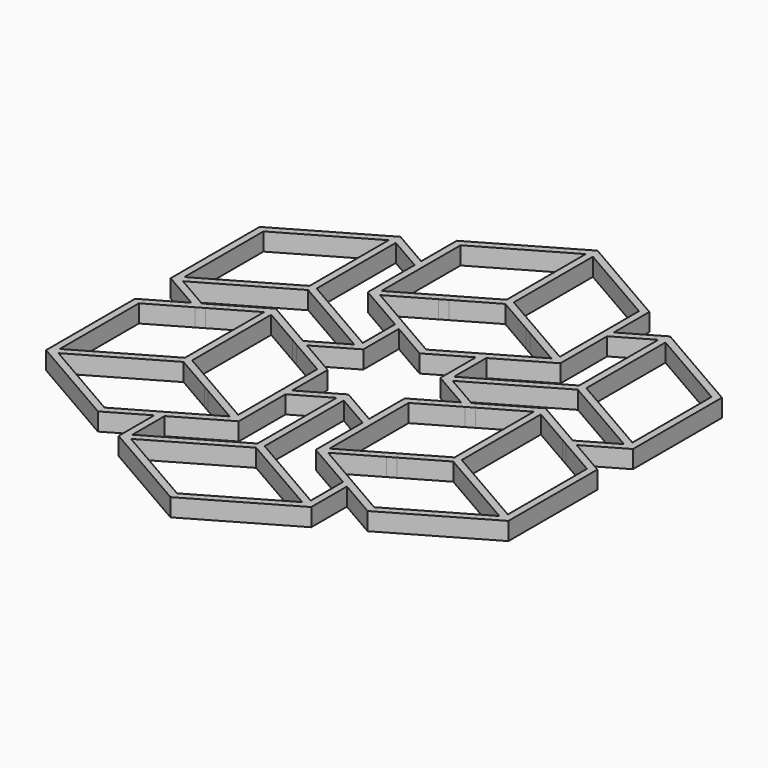
from build123d import *

# Parameters (mm, degrees)
F1_DEPTH = 2


# Not quite as in the source:
# - a feature names something its author has since deleted; it is built from what else it names


with BuildPart() as f1:
    # F0 (on Top) → F1 (new body)
    with BuildSketch(Plane.XY):
        Polygon((-15.1554445662, 3.75), (-20.8506350946, 0.4618802154), (-20.0506350946, 0), (-15.5554445662, 2.5952994616), (-15.5554445662, -2.5952994616), (-15.1554445662, -2.8262395693), (-14.7554445662, -2.5952994616), (-14.7554445662, 2.5952994616), (-10.2602540378, 0), (-9.4602540378, 0.4618802154), align=None)
        Polygon((-15.1554445662, -21.25), (-10.8253175473, -18.75), (-10.8253175473, -17.8262395693), (-15.1554445662, -20.3262395693), (-24.7807621135, -14.7690598923), (-15.1554445662, -9.2118802154), (-10.8253175473, -11.7118802154), (-10.8253175473, -11.25), (-10.4253175473, -11.0190598923), (-14.7554445662, -8.5190598923), (-14.7554445662, -3.5190598923), (-15.1554445662, -3.75), (-15.5554445662, -3.5190598923), (-15.5554445662, -8.5190598923), (-25.1807621135, -14.0762395693), (-25.1807621135, -2.9618802154), (-20.8506350946, -0.4618802154), (-21.6506350946, 0), (-25.9807621135, -2.5), (-25.9807621135, -15), align=None)
        Polygon((-10.0253175473, -17.3643593539), (-10.0253175473, -18.2881197846), (-4.3301270189, -15), (-4.3301270189, -8.4237604307), (-5.1301270189, -8.8856406461), (-5.1301270189, -14.0762395693), (-9.6253175473, -11.4809401077), (-10.0253175473, -11.7118802154), (-10.0253175473, -12.1737604307), (-5.5301270189, -14.7690598923), align=None)
        Polygon((-5.1301270189, -7.9618802154), (-4.3301270189, -7.5), (-4.3301270189, -2.5), (-8.6602540378, 0), (-9.4602540378, -0.4618802154), (-5.1301270189, -2.9618802154), align=None)
        Polygon((-15.1554445662, -3.75), (-14.7554445662, -3.5190598923), (-14.7554445662, -2.5952994616), (-15.1554445662, -2.8262395693), (-15.5554445662, -2.5952994616), (-15.5554445662, -3.5190598923), align=None)
        Polygon((-20.8506350946, 0.4618802154), (-21.6506350946, 0), (-20.8506350946, -0.4618802154), (-20.0506350946, 0), align=None)
        Polygon((-9.4602540378, -0.4618802154), (-8.6602540378, 0), (-9.4602540378, 0.4618802154), (-10.2602540378, 0), align=None)
        Polygon((-25.9807621135, 2.5), (-21.6506350946, 0), (-20.8506350946, 0.4618802154), (-24.7807621135, 2.7309401077), (-15.1554445662, 8.2881197846), (-5.5301270189, 2.7309401077), (-9.4602540378, 0.4618802154), (-8.6602540378, 0), (-4.3301270189, 2.5), (-4.3301270189, 7.5), (-5.1301270189, 7.9618802154), (-5.1301270189, 3.4237604307), (-14.7554445662, 8.9809401077), (-14.7554445662, 20.0952994616), (-10.8253175473, 17.8262395693), (-10.8253175473, 18.75), (-15.1554445662, 21.25), (-25.9807621135, 15), align=None)
        Polygon((-15.5554445662, 8.9809401077), (-25.1807621135, 3.4237604307), (-25.1807621135, 14.5381197846), (-15.5554445662, 20.0952994616), align=None, mode=Mode.SUBTRACT)
        Polygon((-5.1301270189, -8.8856406461), (-4.3301270189, -8.4237604307), (-4.3301270189, -7.5), (-5.1301270189, -7.9618802154), align=None)
        Polygon((-10.8253175473, -11.25), (-10.8253175473, -11.7118802154), (-10.0253175473, -12.1737604307), (-10.0253175473, -11.7118802154), (-9.6253175473, -11.4809401077), (-10.4253175473, -11.0190598923), align=None)
        Polygon((-10.8253175473, -23.75), (0, -30), (10.8253175473, -23.75), (10.8253175473, -18.75), (10.0253175473, -18.2881197846), (10.0253175473, -22.8262395693), (0.4, -17.2690598923), (0.4, -6.1547005384), (4.3301270189, -8.4237604307), (4.3301270189, -7.5), (0, -5), (-4.3301270189, -7.5), (-4.3301270189, -8.4237604307), (-0.4, -6.1547005384), (-0.4, -17.2690598923), (-10.0253175473, -22.8262395693), (-10.0253175473, -18.2881197846), (-10.8253175473, -18.75), align=None)
        Polygon((0, -17.9618802154), (9.6253175473, -23.5190598923), (0, -29.0762395693), (-9.6253175473, -23.5190598923), align=None, mode=Mode.SUBTRACT)
        Polygon((-10.8253175473, -17.8262395693), (-10.8253175473, -18.75), (-10.0253175473, -18.2881197846), (-10.0253175473, -17.3643593539), align=None)
        Polygon((-10.8253175473, 11.25), (-5.1301270189, 7.9618802154), (-5.1301270189, 8.8856406461), (-9.6253175473, 11.4809401077), (-5.1301270189, 14.0762395693), (-5.1301270189, 14.5381197846), (-5.5301270189, 14.7690598923), (-10.0253175473, 12.1737604307), (-10.0253175473, 17.3643593539), (-10.8253175473, 17.8262395693), align=None)
        Polygon((-5.1301270189, 7.9618802154), (-4.3301270189, 7.5), (-4.3301270189, 8.4237604307), (-5.1301270189, 8.8856406461), align=None)
        Polygon((-10.0253175473, 18.2881197846), (-10.8253175473, 18.75), (-10.8253175473, 17.8262395693), (-10.0253175473, 17.3643593539), align=None)
        Polygon((-5.1301270189, 14.0762395693), (-4.3301270189, 14.5381197846), (-4.3301270189, 15), (-4.7301270189, 15.2309401077), (-5.5301270189, 14.7690598923), (-5.1301270189, 14.5381197846), align=None)
        Polygon((-10.8253175473, 23.75), (-10.8253175473, 18.75), (-10.0253175473, 18.2881197846), (-10.0253175473, 23.2881197846), (-0.4, 28.8452994616), (-0.4, 17.7309401077), (-4.7301270189, 15.2309401077), (-4.3301270189, 15), (-4.3301270189, 14.5381197846), (0, 17.0381197846), (4.3301270189, 14.5381197846), (4.3301270189, 15), (4.7301270189, 15.2309401077), (0.4, 17.7309401077), (0.4, 28.8452994616), (10.0253175473, 23.2881197846), (10.0253175473, 18.2881197846), (10.8253175473, 18.75), (10.8253175473, 23.75), (0, 30), align=None)
        Polygon((-4.3301270189, 8.4237604307), (-4.3301270189, 7.5), (0, 5), (4.3301270189, 7.5), (4.3301270189, 8.4237604307), (0, 5.9237604307), align=None)
        Polygon((4.3301270189, 8.4237604307), (4.3301270189, 7.5), (5.1301270189, 7.9618802154), (5.1301270189, 8.8856406461), align=None)
        Polygon((10.8253175473, 11.25), (10.8253175473, 17.8262395693), (10.0253175473, 17.3643593539), (10.0253175473, 12.1737604307), (5.5301270189, 14.7690598923), (5.1301270189, 14.5381197846), (5.1301270189, 14.0762395693), (9.6253175473, 11.4809401077), (5.1301270189, 8.8856406461), (5.1301270189, 7.9618802154), align=None)
        Polygon((5.5301270189, 14.7690598923), (4.7301270189, 15.2309401077), (4.3301270189, 15), (4.3301270189, 14.5381197846), (5.1301270189, 14.0762395693), (5.1301270189, 14.5381197846), align=None)
        Polygon((20.8506350946, 0.4618802154), (21.6506350946, 0), (25.9807621135, 2.5), (25.9807621135, 15), (15.1554445662, 21.25), (10.8253175473, 18.75), (10.8253175473, 17.8262395693), (14.7554445662, 20.0952994616), (14.7554445662, 8.9809401077), (5.1301270189, 3.4237604307), (5.1301270189, 7.9618802154), (4.3301270189, 7.5), (4.3301270189, 2.5), (8.6602540378, 0), (9.4602540378, 0.4618802154), (5.5301270189, 2.7309401077), (15.1554445662, 8.2881197846), (24.7807621135, 2.7309401077), align=None)
        Polygon((15.5554445662, 8.9809401077), (15.5554445662, 20.0952994616), (25.1807621135, 14.5381197846), (25.1807621135, 3.4237604307), align=None, mode=Mode.SUBTRACT)
        Polygon((10.8253175473, 17.8262395693), (10.8253175473, 18.75), (10.0253175473, 18.2881197846), (10.0253175473, 17.3643593539), align=None)
        Polygon((9.4602540378, 0.4618802154), (8.6602540378, 0), (9.4602540378, -0.4618802154), (10.2602540378, 0), align=None)
        Polygon((20.0506350946, 0), (20.8506350946, 0.4618802154), (15.1554445662, 3.75), (9.4602540378, 0.4618802154), (10.2602540378, 0), (14.7554445662, 2.5952994616), (14.7554445662, -2.5952994616), (15.1554445662, -2.8262395693), (15.5554445662, -2.5952994616), (15.5554445662, 2.5952994616), align=None)
        Polygon((14.7554445662, -2.5952994616), (14.7554445662, -3.5190598923), (15.1554445662, -3.75), (15.5554445662, -3.5190598923), (15.5554445662, -2.5952994616), (15.1554445662, -2.8262395693), align=None)
        Polygon((20.8506350946, -0.4618802154), (21.6506350946, 0), (20.8506350946, 0.4618802154), (20.0506350946, 0), align=None)
        Polygon((10.8253175473, -17.8262395693), (10.8253175473, -18.75), (15.1554445662, -21.25), (25.9807621135, -15), (25.9807621135, -2.5), (21.6506350946, 0), (20.8506350946, -0.4618802154), (25.1807621135, -2.9618802154), (25.1807621135, -14.0762395693), (15.5554445662, -8.5190598923), (15.5554445662, -3.5190598923), (15.1554445662, -3.75), (14.7554445662, -3.5190598923), (14.7554445662, -8.5190598923), (10.4253175473, -11.0190598923), (10.8253175473, -11.25), (10.8253175473, -11.7118802154), (15.1554445662, -9.2118802154), (24.7807621135, -14.7690598923), (15.1554445662, -20.3262395693), align=None)
        Polygon((4.3301270189, -2.5), (4.3301270189, -7.5), (5.1301270189, -7.9618802154), (5.1301270189, -2.9618802154), (9.4602540378, -0.4618802154), (8.6602540378, 0), align=None)
        Polygon((4.3301270189, -7.5), (4.3301270189, -8.4237604307), (5.1301270189, -8.8856406461), (5.1301270189, -7.9618802154), align=None)
        Polygon((4.3301270189, -15), (10.0253175473, -18.2881197846), (10.0253175473, -17.3643593539), (5.5301270189, -14.7690598923), (10.0253175473, -12.1737604307), (10.0253175473, -11.7118802154), (9.6253175473, -11.4809401077), (5.1301270189, -14.0762395693), (5.1301270189, -8.8856406461), (4.3301270189, -8.4237604307), align=None)
        Polygon((10.0253175473, -18.2881197846), (10.8253175473, -18.75), (10.8253175473, -17.8262395693), (10.0253175473, -17.3643593539), align=None)
        Polygon((10.0253175473, -12.1737604307), (10.8253175473, -11.7118802154), (10.8253175473, -11.25), (10.4253175473, -11.0190598923), (9.6253175473, -11.4809401077), (10.0253175473, -11.7118802154), align=None)
    extrude(amount=F1_DEPTH)


solid = f1.part
